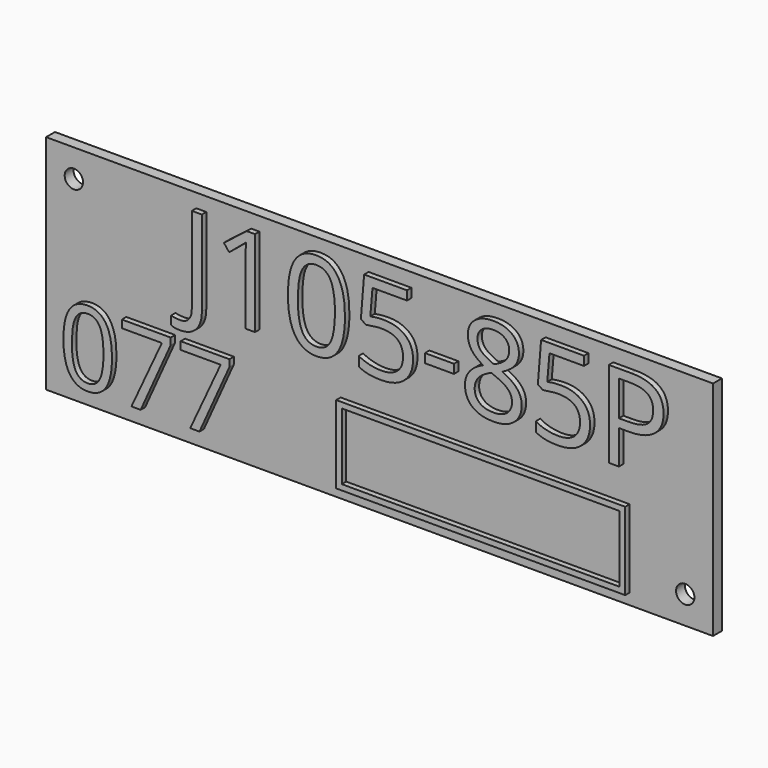
from build123d import *

# Parameters (mm, degrees)
F0_W         = 120
F0_H         = 40
F1_DEPTH     = 2
F3_D         = 3.3
F4_TEXT_SIZE = 21.733388673
F5_DEPTH     = 1
F6_TEXT_SIZE = 18.5054667028
F7_DEPTH     = 1
F8_W         = 52
F8_H         = 14
F8_W_2       = 49.99999962
F8_H_2       = 11.99999962
F9_DEPTH     = 1


# Not quite as in the source:
# - Text() gives the source's letters only with a copy of the font that has no kerning and outlines rounded to 1/6400 em; it was checked with that copy


with BuildPart() as f1:
    # F0 (on Front) → F1 (new body)
    with BuildSketch(Plane.XZ):
        Rectangle(F0_W, F0_H)
    extrude(amount=F1_DEPTH)

    # F3 (through all)
    with Locations(Plane.XZ.offset(2)):
        with Locations((-55, 15), (55, -15)):
            Hole(F3_D / 2)

    # F4 (on face) → F5 (join)
    with BuildSketch(Plane.XZ.offset(2)):
        with Locations((-35, 2)):
            Text('J105-85P', F4_TEXT_SIZE, font='Open Sans', text_align=(TextAlign.LEFT, TextAlign.BOTTOM))
    extrude(amount=F5_DEPTH)

    # F6 (on face) → F7 (join)
    with BuildSketch(Plane.XZ.offset(2)):
        with Locations((-57, -17)):
            Text('077', F6_TEXT_SIZE, font='Open Sans', text_align=(TextAlign.LEFT, TextAlign.BOTTOM))
    extrude(amount=F7_DEPTH)

    # F8 (on face) → F9 (join)
    with BuildSketch(Plane.XZ.offset(2)):
        with Locations((19, -11)):
            Rectangle(F8_W, F8_H)
        with Locations((19, -11)):
            Rectangle(F8_W_2, F8_H_2, mode=Mode.SUBTRACT)
    extrude(amount=F9_DEPTH)


solid = f1.part
